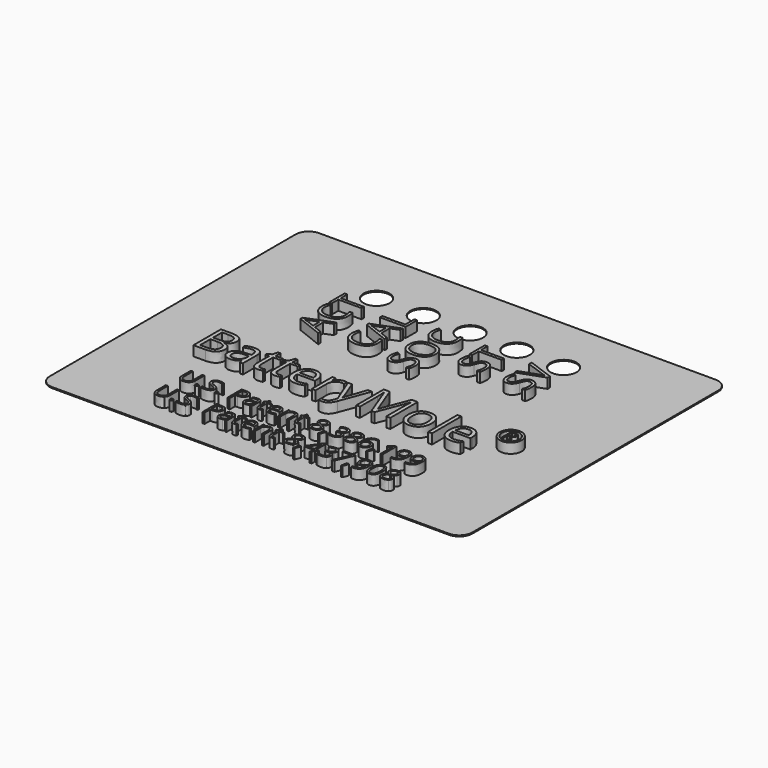
from build123d import *

# Parameters (mm, degrees)
F0_R           = 1.5
F2_DEPTH       = 0.127
F1_R           = 1.27
F1_R_2         = 1.016
F1_TEXT_SIZE   = 4.1666666667
F1_TEXT_SIZE_2 = 5.5555555556
F1_TEXT_SIZE_3 = 2.0717814957
F1_TEXT_SIZE_4 = 2.8222222222
F3_DEPTH       = 1.27


# Not quite as in the source:
# - Text() gives the source's letters only with a copy of the font that has no kerning and outlines rounded to 1/6400 em; it was checked with that copy


with BuildPart() as f2:
    # F0 (on Top) → F2 (new body)
    with BuildSketch(Plane.XY):
        with BuildLine():
            Line((47.3, 38.5), (1.5, 38.5))
            ThreePointArc((1.5, 38.5), (0.4393398282, 38.0606601718), (0, 37))
            Line((0, 37), (0, 1.5))
            ThreePointArc((0, 1.5), (0.4393398282, 0.4393398282), (1.5, 0))
            Line((1.5, 0), (47.3, 0))
            ThreePointArc((47.3, 0), (48.3606601718, 0.4393398282), (48.8, 1.5))
            Line((48.8, 1.5), (48.8, 37))
            ThreePointArc((48.8, 37), (48.3606601718, 38.0606601718), (47.3, 38.5))
        make_face()
        with Locations((13.5, 31.8)):
            Circle(F0_R, mode=Mode.SUBTRACT)
        with Locations((18.9, 31.8)):
            Circle(F0_R, mode=Mode.SUBTRACT)
        with Locations((24.3, 31.8)):
            Circle(F0_R, mode=Mode.SUBTRACT)
        with Locations((29.7, 31.8)):
            Circle(F0_R, mode=Mode.SUBTRACT)
        with Locations((35.1, 31.8)):
            Circle(F0_R, mode=Mode.SUBTRACT)
    extrude(amount=F2_DEPTH)

    # F1 (on Top) → F3 (join)
    with BuildSketch(Plane.XY):
        with Locations((41.1306089235, 16.6292472288)):
            Circle(F1_R)
        with Locations((41.1306089235, 16.6292472288)):
            Circle(F1_R_2, mode=Mode.SUBTRACT)
        with BuildLine():
            add(Edge.make_bspline(
                [(36.4412881944, 3.9645432287), (36.4412881944, 3.4419911453), (36.2765850694, 3.1842428814)],
                knots=[0, 0, 0, 1, 1, 1], degree=2))
            add(Edge.make_bspline(
                [(36.2710729167, 4.7347012148), (36.4412881944, 4.4685744787), (36.4412881944, 3.9645432287)],
                knots=[0, 0, 0, 1, 1, 1], degree=2))
            add(Edge.make_bspline(
                [(35.7727743056, 5.0008279509), (36.1008576389, 5.0008279509), (36.2710729167, 4.7347012148)],
                knots=[0, 0, 0, 1, 1, 1], degree=2))
            add(Edge.make_bspline(
                [(35.2727118056, 4.7457255203), (35.4367534722, 5.0008279509), (35.7727743056, 5.0008279509)],
                knots=[0, 0, 0, 1, 1, 1], degree=2))
            add(Edge.make_bspline(
                [(35.1086701389, 3.9645432287), (35.1086701389, 4.4906230898), (35.2727118056, 4.7457255203)],
                knots=[0, 0, 0, 1, 1, 1], degree=2))
            add(Edge.make_bspline(
                [(35.2782239583, 3.1904164925), (35.1086701389, 3.4543383675), (35.1086701389, 3.9645432287)],
                knots=[0, 0, 0, 1, 1, 1], degree=2))
            add(Edge.make_bspline(
                [(35.7727743056, 2.9264946175), (35.4477777778, 2.9264946175), (35.2782239583, 3.1904164925)],
                knots=[0, 0, 0, 1, 1, 1], degree=2))
            add(Edge.make_bspline(
                [(36.2765850694, 3.1842428814), (36.1118819444, 2.9264946175), (35.7727743056, 2.9264946175)],
                knots=[0, 0, 0, 1, 1, 1], degree=2))
        make_face()
        with BuildLine():
            add(Edge.make_bspline(
                [(35.3401805556, 3.9645432287), (35.3401805556, 3.5248939231), (35.4435885417, 3.324251562)],
                knots=[0, 0, 0, 1, 1, 1], degree=2))
            add(Edge.make_bspline(
                [(35.4435885417, 4.6032914925), (35.3401805556, 4.4041925342), (35.3401805556, 3.9645432287)],
                knots=[0, 0, 0, 1, 1, 1], degree=2))
            add(Edge.make_bspline(
                [(35.7727743056, 4.8023904509), (35.5469965278, 4.8023904509), (35.4435885417, 4.6032914925)],
                knots=[0, 0, 0, 1, 1, 1], degree=2))
            add(Edge.make_bspline(
                [(36.1041649306, 4.6004251731), (36.0016388889, 4.8023904509), (35.7727743056, 4.8023904509)],
                knots=[0, 0, 0, 1, 1, 1], degree=2))
            add(Edge.make_bspline(
                [(36.2066909722, 3.9645432287), (36.2066909722, 4.3984598953), (36.1041649306, 4.6004251731)],
                knots=[0, 0, 0, 1, 1, 1], degree=2))
            add(Edge.make_bspline(
                [(36.1041649306, 3.3268973953), (36.2066909722, 3.5301855898), (36.2066909722, 3.9645432287)],
                knots=[0, 0, 0, 1, 1, 1], degree=2))
            add(Edge.make_bspline(
                [(35.7727743056, 3.1236092009), (36.0016388889, 3.1236092009), (36.1041649306, 3.3268973953)],
                knots=[0, 0, 0, 1, 1, 1], degree=2))
            add(Edge.make_bspline(
                [(35.4435885417, 3.324251562), (35.5469965278, 3.1236092009), (35.7727743056, 3.1236092009)],
                knots=[0, 0, 0, 1, 1, 1], degree=2))
        make_face(mode=Mode.SUBTRACT)
        with BuildLine():
            add(Edge.make_bspline(
                [(37.3862916667, 4.9977411453), (37.6618993056, 4.9977411453), (37.8230746528, 4.8696387148)],
                knots=[0, 0, 0, 1, 1, 1], degree=2))
            add(Edge.make_bspline(
                [(36.9528159722, 4.8676543398), (37.1146527778, 4.9977411453), (37.3862916667, 4.9977411453)],
                knots=[0, 0, 0, 1, 1, 1], degree=2))
            add(Edge.make_bspline(
                [(36.7909791667, 4.5184043398), (36.7909791667, 4.7375675342), (36.9528159722, 4.8676543398)],
                knots=[0, 0, 0, 1, 1, 1], degree=2))
            add(Edge.make_bspline(
                [(36.8736614583, 4.2392689231), (36.7909791667, 4.364064062), (36.7909791667, 4.5184043398)],
                knots=[0, 0, 0, 1, 1, 1], degree=2))
            add(Edge.make_bspline(
                [(37.1464027778, 4.0073175342), (36.95634375, 4.1144737842), (36.8736614583, 4.2392689231)],
                knots=[0, 0, 0, 1, 1, 1], degree=2))
            add(Edge.make_bspline(
                [(36.7248333333, 3.4684494787), (36.7248333333, 3.8141717009), (37.1464027778, 4.0073175342)],
                knots=[0, 0, 0, 1, 1, 1], degree=2))
            add(Edge.make_bspline(
                [(36.8985763889, 3.0678262148), (36.7248333333, 3.209157812), (36.7248333333, 3.4684494787)],
                knots=[0, 0, 0, 1, 1, 1], degree=2))
            add(Edge.make_bspline(
                [(37.3946701389, 2.9264946175), (37.0723194444, 2.9264946175), (36.8985763889, 3.0678262148)],
                knots=[0, 0, 0, 1, 1, 1], degree=2))
            add(Edge.make_bspline(
                [(37.8740069444, 3.076204687), (37.6989409722, 2.9264946175), (37.3946701389, 2.9264946175)],
                knots=[0, 0, 0, 1, 1, 1], degree=2))
            add(Edge.make_bspline(
                [(38.0490729167, 3.4763869787), (38.0490729167, 3.2259147564), (37.8740069444, 3.076204687)],
                knots=[0, 0, 0, 1, 1, 1], degree=2))
            add(Edge.make_bspline(
                [(37.9456649306, 3.7749251731), (38.0490729167, 3.6461612842), (38.0490729167, 3.4763869787)],
                knots=[0, 0, 0, 1, 1, 1], degree=2))
            add(Edge.make_bspline(
                [(37.5970763889, 4.0209876731), (37.8422569444, 3.903689062), (37.9456649306, 3.7749251731)],
                knots=[0, 0, 0, 1, 1, 1], degree=2))
            add(Edge.make_bspline(
                [(37.8920868056, 4.2441196175), (37.7999236111, 4.1215293398), (37.5970763889, 4.0209876731)],
                knots=[0, 0, 0, 1, 1, 1], degree=2))
            add(Edge.make_bspline(
                [(37.98425, 4.5157585064), (37.98425, 4.3667098953), (37.8920868056, 4.2441196175)],
                knots=[0, 0, 0, 1, 1, 1], degree=2))
            add(Edge.make_bspline(
                [(37.8230746528, 4.8696387148), (37.98425, 4.7415362842), (37.98425, 4.5157585064)],
                knots=[0, 0, 0, 1, 1, 1], degree=2))
        make_face()
        with BuildLine():
            add(Edge.make_bspline(
                [(36.9510520833, 3.4627168398), (36.9510520833, 3.2973522564), (37.0659253472, 3.2049685759)],
                knots=[0, 0, 0, 1, 1, 1], degree=2))
            add(Edge.make_bspline(
                [(37.0432152778, 3.7184807287), (36.9510520833, 3.6117654509), (36.9510520833, 3.4627168398)],
                knots=[0, 0, 0, 1, 1, 1], degree=2))
            add(Edge.make_bspline(
                [(37.3408715278, 3.9133904509), (37.1353784722, 3.8251960064), (37.0432152778, 3.7184807287)],
                knots=[0, 0, 0, 1, 1, 1], degree=2))
            add(Edge.make_bspline(
                [(37.7156979167, 3.7114251731), (37.6081006944, 3.8154946175), (37.3408715278, 3.9133904509)],
                knots=[0, 0, 0, 1, 1, 1], degree=2))
            add(Edge.make_bspline(
                [(37.8232951389, 3.4737411453), (37.8232951389, 3.6073557287), (37.7156979167, 3.7114251731)],
                knots=[0, 0, 0, 1, 1, 1], degree=2))
            add(Edge.make_bspline(
                [(37.7088628472, 3.209157812), (37.8232951389, 3.3057307287), (37.8232951389, 3.4737411453)],
                knots=[0, 0, 0, 1, 1, 1], degree=2))
            add(Edge.make_bspline(
                [(37.3889375, 3.1125848953), (37.5944305556, 3.1125848953), (37.7088628472, 3.209157812)],
                knots=[0, 0, 0, 1, 1, 1], degree=2))
            add(Edge.make_bspline(
                [(37.0659253472, 3.2049685759), (37.1807986111, 3.1125848953), (37.3889375, 3.1125848953)],
                knots=[0, 0, 0, 1, 1, 1], degree=2))
        make_face(mode=Mode.SUBTRACT)
        with BuildLine():
            add(Edge.make_bspline(
                [(37.3836458333, 4.8120918398), (37.2112256944, 4.8120918398), (37.1133298611, 4.7294095481)],
                knots=[0, 0, 0, 1, 1, 1], degree=2))
            add(Edge.make_bspline(
                [(37.6585920139, 4.7300710064), (37.5587118056, 4.8120918398), (37.3836458333, 4.8120918398)],
                knots=[0, 0, 0, 1, 1, 1], degree=2))
            add(Edge.make_bspline(
                [(37.7584722222, 4.5087029509), (37.7584722222, 4.6480501731), (37.6585920139, 4.7300710064)],
                knots=[0, 0, 0, 1, 1, 1], degree=2))
            add(Edge.make_bspline(
                [(37.6764513889, 4.2868939231), (37.7584722222, 4.3821439231), (37.7584722222, 4.5087029509)],
                knots=[0, 0, 0, 1, 1, 1], degree=2))
            add(Edge.make_bspline(
                [(37.3973159722, 4.1091821175), (37.5944305556, 4.1916439231), (37.6764513889, 4.2868939231)],
                knots=[0, 0, 0, 1, 1, 1], degree=2))
            add(Edge.make_bspline(
                [(37.0967934028, 4.2910831592), (37.1781527778, 4.2000223953), (37.3973159722, 4.1091821175)],
                knots=[0, 0, 0, 1, 1, 1], degree=2))
            add(Edge.make_bspline(
                [(37.0154340278, 4.5087029509), (37.0154340278, 4.3821439231), (37.0967934028, 4.2910831592)],
                knots=[0, 0, 0, 1, 1, 1], degree=2))
            add(Edge.make_bspline(
                [(37.1133298611, 4.7294095481), (37.0154340278, 4.6467272564), (37.0154340278, 4.5087029509)],
                knots=[0, 0, 0, 1, 1, 1], degree=2))
        make_face(mode=Mode.SUBTRACT)
        with BuildLine():
            add(Edge.make_bspline(
                [(26.3214166667, 4.9977411453), (26.5970243056, 4.9977411453), (26.7581996528, 4.8696387148)],
                knots=[0, 0, 0, 1, 1, 1], degree=2))
            add(Edge.make_bspline(
                [(25.8879409722, 4.8676543398), (26.0497777778, 4.9977411453), (26.3214166667, 4.9977411453)],
                knots=[0, 0, 0, 1, 1, 1], degree=2))
            add(Edge.make_bspline(
                [(25.7261041667, 4.5184043398), (25.7261041667, 4.7375675342), (25.8879409722, 4.8676543398)],
                knots=[0, 0, 0, 1, 1, 1], degree=2))
            add(Edge.make_bspline(
                [(25.8087864583, 4.2392689231), (25.7261041667, 4.364064062), (25.7261041667, 4.5184043398)],
                knots=[0, 0, 0, 1, 1, 1], degree=2))
            add(Edge.make_bspline(
                [(26.0815277778, 4.0073175342), (25.89146875, 4.1144737842), (25.8087864583, 4.2392689231)],
                knots=[0, 0, 0, 1, 1, 1], degree=2))
            add(Edge.make_bspline(
                [(25.6599583333, 3.4684494787), (25.6599583333, 3.8141717009), (26.0815277778, 4.0073175342)],
                knots=[0, 0, 0, 1, 1, 1], degree=2))
            add(Edge.make_bspline(
                [(25.8337013889, 3.0678262148), (25.6599583333, 3.209157812), (25.6599583333, 3.4684494787)],
                knots=[0, 0, 0, 1, 1, 1], degree=2))
            add(Edge.make_bspline(
                [(26.3297951389, 2.9264946175), (26.0074444444, 2.9264946175), (25.8337013889, 3.0678262148)],
                knots=[0, 0, 0, 1, 1, 1], degree=2))
            add(Edge.make_bspline(
                [(26.8091319444, 3.076204687), (26.6340659722, 2.9264946175), (26.3297951389, 2.9264946175)],
                knots=[0, 0, 0, 1, 1, 1], degree=2))
            add(Edge.make_bspline(
                [(26.9841979167, 3.4763869787), (26.9841979167, 3.2259147564), (26.8091319444, 3.076204687)],
                knots=[0, 0, 0, 1, 1, 1], degree=2))
            add(Edge.make_bspline(
                [(26.8807899306, 3.7749251731), (26.9841979167, 3.6461612842), (26.9841979167, 3.4763869787)],
                knots=[0, 0, 0, 1, 1, 1], degree=2))
            add(Edge.make_bspline(
                [(26.5322013889, 4.0209876731), (26.7773819444, 3.903689062), (26.8807899306, 3.7749251731)],
                knots=[0, 0, 0, 1, 1, 1], degree=2))
            add(Edge.make_bspline(
                [(26.8272118056, 4.2441196175), (26.7350486111, 4.1215293398), (26.5322013889, 4.0209876731)],
                knots=[0, 0, 0, 1, 1, 1], degree=2))
            add(Edge.make_bspline(
                [(26.919375, 4.5157585064), (26.919375, 4.3667098953), (26.8272118056, 4.2441196175)],
                knots=[0, 0, 0, 1, 1, 1], degree=2))
            add(Edge.make_bspline(
                [(26.7581996528, 4.8696387148), (26.919375, 4.7415362842), (26.919375, 4.5157585064)],
                knots=[0, 0, 0, 1, 1, 1], degree=2))
        make_face()
        with BuildLine():
            add(Edge.make_bspline(
                [(25.8861770833, 3.4627168398), (25.8861770833, 3.2973522564), (26.0010503472, 3.2049685759)],
                knots=[0, 0, 0, 1, 1, 1], degree=2))
            add(Edge.make_bspline(
                [(25.9783402778, 3.7184807287), (25.8861770833, 3.6117654509), (25.8861770833, 3.4627168398)],
                knots=[0, 0, 0, 1, 1, 1], degree=2))
            add(Edge.make_bspline(
                [(26.2759965278, 3.9133904509), (26.0705034722, 3.8251960064), (25.9783402778, 3.7184807287)],
                knots=[0, 0, 0, 1, 1, 1], degree=2))
            add(Edge.make_bspline(
                [(26.6508229167, 3.7114251731), (26.5432256944, 3.8154946175), (26.2759965278, 3.9133904509)],
                knots=[0, 0, 0, 1, 1, 1], degree=2))
            add(Edge.make_bspline(
                [(26.7584201389, 3.4737411453), (26.7584201389, 3.6073557287), (26.6508229167, 3.7114251731)],
                knots=[0, 0, 0, 1, 1, 1], degree=2))
            add(Edge.make_bspline(
                [(26.6439878472, 3.209157812), (26.7584201389, 3.3057307287), (26.7584201389, 3.4737411453)],
                knots=[0, 0, 0, 1, 1, 1], degree=2))
            add(Edge.make_bspline(
                [(26.3240625, 3.1125848953), (26.5295555556, 3.1125848953), (26.6439878472, 3.209157812)],
                knots=[0, 0, 0, 1, 1, 1], degree=2))
            add(Edge.make_bspline(
                [(26.0010503472, 3.2049685759), (26.1159236111, 3.1125848953), (26.3240625, 3.1125848953)],
                knots=[0, 0, 0, 1, 1, 1], degree=2))
        make_face(mode=Mode.SUBTRACT)
        with BuildLine():
            add(Edge.make_bspline(
                [(26.3187708333, 4.8120918398), (26.1463506944, 4.8120918398), (26.0484548611, 4.7294095481)],
                knots=[0, 0, 0, 1, 1, 1], degree=2))
            add(Edge.make_bspline(
                [(26.5937170139, 4.7300710064), (26.4938368056, 4.8120918398), (26.3187708333, 4.8120918398)],
                knots=[0, 0, 0, 1, 1, 1], degree=2))
            add(Edge.make_bspline(
                [(26.6935972222, 4.5087029509), (26.6935972222, 4.6480501731), (26.5937170139, 4.7300710064)],
                knots=[0, 0, 0, 1, 1, 1], degree=2))
            add(Edge.make_bspline(
                [(26.6115763889, 4.2868939231), (26.6935972222, 4.3821439231), (26.6935972222, 4.5087029509)],
                knots=[0, 0, 0, 1, 1, 1], degree=2))
            add(Edge.make_bspline(
                [(26.3324409722, 4.1091821175), (26.5295555556, 4.1916439231), (26.6115763889, 4.2868939231)],
                knots=[0, 0, 0, 1, 1, 1], degree=2))
            add(Edge.make_bspline(
                [(26.0319184028, 4.2910831592), (26.1132777778, 4.2000223953), (26.3324409722, 4.1091821175)],
                knots=[0, 0, 0, 1, 1, 1], degree=2))
            add(Edge.make_bspline(
                [(25.9505590278, 4.5087029509), (25.9505590278, 4.3821439231), (26.0319184028, 4.2910831592)],
                knots=[0, 0, 0, 1, 1, 1], degree=2))
            add(Edge.make_bspline(
                [(26.0484548611, 4.7294095481), (25.9505590278, 4.6467272564), (25.9505590278, 4.5087029509)],
                knots=[0, 0, 0, 1, 1, 1], degree=2))
        make_face(mode=Mode.SUBTRACT)
        with Locations(Location((36.6, 24.262890625), (0, 0, 90))):
            Text('SV', F1_TEXT_SIZE, font='Open Sans', text_align=(TextAlign.LEFT, TextAlign.BOTTOM))
        with Locations(Location((25.8, 20.993359375), (0, 0, 90))):
            Text('SOC', F1_TEXT_SIZE, font='Open Sans', text_align=(TextAlign.LEFT, TextAlign.BOTTOM))
        with Locations((7.1502256944, 12.6292472288)):
            Text('BatteryMole', F1_TEXT_SIZE_2, font='Open Sans', text_align=(TextAlign.LEFT, TextAlign.BOTTOM))
        with BuildLine():
            add(Edge.make_bspline(
                [(34.8167465278, 4.1091821175), (34.8167465278, 2.9264946175), (33.9017291667, 2.9264946175)],
                knots=[0, 0, 0, 1, 1, 1], degree=2))
            add(Edge.make_bspline(
                [(34.7340642361, 4.5852116314), (34.8167465278, 4.3834668398), (34.8167465278, 4.1091821175)],
                knots=[0, 0, 0, 1, 1, 1], degree=2))
            add(Edge.make_bspline(
                [(34.497703125, 4.8923487842), (34.6513819444, 4.7869564231), (34.7340642361, 4.5852116314)],
                knots=[0, 0, 0, 1, 1, 1], degree=2))
            add(Edge.make_bspline(
                [(34.13853125, 4.9977411453), (34.3440243056, 4.9977411453), (34.497703125, 4.8923487842)],
                knots=[0, 0, 0, 1, 1, 1], degree=2))
            add(Edge.make_bspline(
                [(33.676171875, 4.8158401037), (33.8518993056, 4.9977411453), (34.13853125, 4.9977411453)],
                knots=[0, 0, 0, 1, 1, 1], degree=2))
            add(Edge.make_bspline(
                [(33.5004444444, 4.3199668398), (33.5004444444, 4.633939062), (33.676171875, 4.8158401037)],
                knots=[0, 0, 0, 1, 1, 1], degree=2))
            add(Edge.make_bspline(
                [(33.6576510417, 3.8734824648), (33.5004444444, 4.0333348953), (33.5004444444, 4.3199668398)],
                knots=[0, 0, 0, 1, 1, 1], degree=2))
            add(Edge.make_bspline(
                [(34.0820868056, 3.7136300342), (33.8148576389, 3.7136300342), (33.6576510417, 3.8734824648)],
                knots=[0, 0, 0, 1, 1, 1], degree=2))
            add(Edge.make_bspline(
                [(34.3645295139, 3.7736022564), (34.2390729167, 3.7136300342), (34.0820868056, 3.7136300342)],
                knots=[0, 0, 0, 1, 1, 1], degree=2))
            add(Edge.make_bspline(
                [(34.5658333333, 3.9477862842), (34.4899861111, 3.8335744787), (34.3645295139, 3.7736022564)],
                knots=[0, 0, 0, 1, 1, 1], degree=2))
            Line((34.5658333333, 3.9477862842), (34.5821493056, 3.9477862842))
            add(Edge.make_bspline(
                [(34.3982638889, 3.320282812), (34.56715625, 3.5248939231), (34.5821493056, 3.9477862842)],
                knots=[0, 0, 0, 1, 1, 1], degree=2))
            add(Edge.make_bspline(
                [(33.8986423611, 3.1156717009), (34.2293715278, 3.1156717009), (34.3982638889, 3.320282812)],
                knots=[0, 0, 0, 1, 1, 1], degree=2))
            add(Edge.make_bspline(
                [(33.6481701389, 3.1513904509), (33.7584131944, 3.1156717009), (33.8986423611, 3.1156717009)],
                knots=[0, 0, 0, 1, 1, 1], degree=2))
            Line((33.6481701389, 3.1513904509), (33.6481701389, 2.9542758675))
            add(Edge.make_bspline(
                [(33.9017291667, 2.9264946175), (33.74165625, 2.9264946175), (33.6481701389, 2.9542758675)],
                knots=[0, 0, 0, 1, 1, 1], degree=2))
        make_face()
        with BuildLine():
            add(Edge.make_bspline(
                [(34.13853125, 4.8023904509), (33.9414166667, 4.8023904509), (33.8340399306, 4.675610937)],
                knots=[0, 0, 0, 1, 1, 1], degree=2))
            add(Edge.make_bspline(
                [(34.370703125, 4.7320553814), (34.2695, 4.8023904509), (34.13853125, 4.8023904509)],
                knots=[0, 0, 0, 1, 1, 1], degree=2))
            add(Edge.make_bspline(
                [(34.5285711806, 4.5391300342), (34.47190625, 4.661720312), (34.370703125, 4.7320553814)],
                knots=[0, 0, 0, 1, 1, 1], degree=2))
            add(Edge.make_bspline(
                [(34.5852361111, 4.2719008675), (34.5852361111, 4.4165397564), (34.5285711806, 4.5391300342)],
                knots=[0, 0, 0, 1, 1, 1], degree=2))
            add(Edge.make_bspline(
                [(34.5246024306, 4.0871335064), (34.5852361111, 4.1753279509), (34.5852361111, 4.2719008675)],
                knots=[0, 0, 0, 1, 1, 1], degree=2))
            add(Edge.make_bspline(
                [(34.3585763889, 3.9480067703), (34.46396875, 3.998939062), (34.5246024306, 4.0871335064)],
                knots=[0, 0, 0, 1, 1, 1], degree=2))
            add(Edge.make_bspline(
                [(34.1275069444, 3.8970744787), (34.2531840278, 3.8970744787), (34.3585763889, 3.9480067703)],
                knots=[0, 0, 0, 1, 1, 1], degree=2))
            add(Edge.make_bspline(
                [(33.8258819444, 4.0106248259), (33.9251006944, 3.8970744787), (34.1275069444, 3.8970744787)],
                knots=[0, 0, 0, 1, 1, 1], degree=2))
            add(Edge.make_bspline(
                [(33.7266631944, 4.3226126731), (33.7266631944, 4.1241751731), (33.8258819444, 4.0106248259)],
                knots=[0, 0, 0, 1, 1, 1], degree=2))
            add(Edge.make_bspline(
                [(33.8340399306, 4.675610937), (33.7266631944, 4.5488314231), (33.7266631944, 4.3226126731)],
                knots=[0, 0, 0, 1, 1, 1], degree=2))
        make_face(mode=Mode.SUBTRACT)
        with Locations(Location((31.2, 24.4764322917), (0, 0, 90))):
            Text('ST', F1_TEXT_SIZE, font='Open Sans', text_align=(TextAlign.LEFT, TextAlign.BOTTOM))
        with Locations(Location((15, 21.4979166667), (0, 0, 90))):
            Text('ACT', F1_TEXT_SIZE, font='Open Sans', text_align=(TextAlign.LEFT, TextAlign.BOTTOM))
        with BuildLine():
            add(Edge.make_bspline(
                [(17.7612638889, 4.3821439231), (17.7612638889, 4.0761092009), (17.5524635417, 3.9114060759)],
                knots=[0, 0, 0, 1, 1, 1], degree=2))
            add(Edge.make_bspline(
                [(17.0063194444, 4.9690779509), (17.7612638889, 4.9690779509), (17.7612638889, 4.3821439231)],
                knots=[0, 0, 0, 1, 1, 1], degree=2))
            Line((17.0063194444, 4.9690779509), (16.4837673611, 4.9690779509))
            Line((16.4837673611, 4.9690779509), (16.4837673611, 2.9542758675))
            Line((16.4837673611, 2.9542758675), (16.7179236111, 2.9542758675))
            Line((16.7179236111, 2.9542758675), (16.7179236111, 3.7467029509))
            Line((16.7179236111, 3.7467029509), (16.9551666667, 3.7467029509))
            add(Edge.make_bspline(
                [(17.5524635417, 3.9114060759), (17.3436631944, 3.7467029509), (16.9551666667, 3.7467029509)],
                knots=[0, 0, 0, 1, 1, 1], degree=2))
        make_face()
        with BuildLine():
            Line((16.9291493056, 3.9477862842), (16.7179236111, 3.9477862842))
            Line((16.7179236111, 3.9477862842), (16.7179236111, 4.7662307287))
            Line((16.7179236111, 4.7662307287), (16.9798611111, 4.7662307287))
            add(Edge.make_bspline(
                [(17.3877604167, 4.6685553814), (17.2567916667, 4.7662307287), (16.9798611111, 4.7662307287)],
                knots=[0, 0, 0, 1, 1, 1], degree=2))
            add(Edge.make_bspline(
                [(17.5187291667, 4.3711196175), (17.5187291667, 4.5708800342), (17.3877604167, 4.6685553814)],
                knots=[0, 0, 0, 1, 1, 1], degree=2))
            add(Edge.make_bspline(
                [(17.3796024306, 4.0483279509), (17.5187291667, 4.1488696175), (17.5187291667, 4.3711196175)],
                knots=[0, 0, 0, 1, 1, 1], degree=2))
            add(Edge.make_bspline(
                [(16.9291493056, 3.9477862842), (17.2404756944, 3.9477862842), (17.3796024306, 4.0483279509)],
                knots=[0, 0, 0, 1, 1, 1], degree=2))
        make_face(mode=Mode.SUBTRACT)
        with Locations(Location((20.4, 21.6971354167), (0, 0, 90))):
            Text('CAL', F1_TEXT_SIZE, font='Open Sans', text_align=(TextAlign.LEFT, TextAlign.BOTTOM))
        Polygon((29.0801388889, 3.4172967009), (29.3791180556, 3.4172967009), (29.3791180556, 3.6254355898), (29.0801388889, 3.6254355898), (29.0801388889, 4.9801022564), (28.8376041667, 4.9801022564), (27.8811354167, 3.6170571175), (27.8811354167, 3.4172967009), (28.8609756944, 3.4172967009), (28.8609756944, 2.9542758675), (29.0801388889, 2.9542758675), align=None)
        with BuildLine():
            Line((28.8609756944, 4.2952723953), (28.8609756944, 3.6254355898))
            Line((28.8609756944, 3.6254355898), (28.11, 3.6254355898))
            Line((28.11, 3.6254355898), (28.7397083333, 4.5210501731))
            add(Edge.make_bspline(
                [(28.8640625, 4.7402133675), (28.7979166667, 4.6079217009), (28.7397083333, 4.5210501731)],
                knots=[0, 0, 0, 1, 1, 1], degree=2))
            Line((28.8640625, 4.7402133675), (28.8750868056, 4.7402133675))
            add(Edge.make_bspline(
                [(28.8609756944, 4.2952723953), (28.8609756944, 4.4923869787), (28.8750868056, 4.7402133675)],
                knots=[0, 0, 0, 1, 1, 1], degree=2))
        make_face(mode=Mode.SUBTRACT)
        with BuildLine():
            Line((19.0317048611, 3.169470312), (19.077125, 2.9542758675))
            Line((19.077125, 2.9542758675), (19.2468993056, 2.9542758675))
            Line((19.2468993056, 2.9542758675), (19.2468993056, 3.9852689231))
            add(Edge.make_bspline(
                [(19.1165920139, 4.3695762148), (19.2468993056, 4.2498522564), (19.2468993056, 3.9852689231)],
                knots=[0, 0, 0, 1, 1, 1], degree=2))
            add(Edge.make_bspline(
                [(18.7164097222, 4.4893001731), (18.9862847222, 4.4893001731), (19.1165920139, 4.3695762148)],
                knots=[0, 0, 0, 1, 1, 1], degree=2))
            add(Edge.make_bspline(
                [(18.4494010417, 4.4549043398), (18.5823541667, 4.4893001731), (18.7164097222, 4.4893001731)],
                knots=[0, 0, 0, 1, 1, 1], degree=2))
            add(Edge.make_bspline(
                [(18.2048819444, 4.360095312), (18.3164479167, 4.4205085064), (18.4494010417, 4.4549043398)],
                knots=[0, 0, 0, 1, 1, 1], degree=2))
            Line((18.2048819444, 4.360095312), (18.2754375, 4.1850293398))
            add(Edge.make_bspline(
                [(18.7022986111, 4.300564062), (18.5135625, 4.300564062), (18.2754375, 4.1850293398)],
                knots=[0, 0, 0, 1, 1, 1], degree=2))
            add(Edge.make_bspline(
                [(18.9470381944, 4.2158973953), (18.87075, 4.300564062), (18.7022986111, 4.300564062)],
                knots=[0, 0, 0, 1, 1, 1], degree=2))
            add(Edge.make_bspline(
                [(19.0233263889, 3.9535189231), (19.0233263889, 4.1312307287), (18.9470381944, 4.2158973953)],
                knots=[0, 0, 0, 1, 1, 1], degree=2))
            Line((19.0233263889, 3.9535189231), (19.0233263889, 3.8595918398))
            Line((19.0233263889, 3.8595918398), (18.7671215278, 3.8512133675))
            add(Edge.make_bspline(
                [(18.0355486111, 3.371876562), (18.0355486111, 3.8291647564), (18.7671215278, 3.8512133675)],
                knots=[0, 0, 0, 1, 1, 1], degree=2))
            add(Edge.make_bspline(
                [(18.1629895833, 3.042470312), (18.0355486111, 3.1584460064), (18.0355486111, 3.371876562)],
                knots=[0, 0, 0, 1, 1, 1], degree=2))
            add(Edge.make_bspline(
                [(18.5148854167, 2.9264946175), (18.2904305556, 2.9264946175), (18.1629895833, 3.042470312)],
                knots=[0, 0, 0, 1, 1, 1], degree=2))
            add(Edge.make_bspline(
                [(18.7955642361, 2.976985937), (18.6833368056, 2.9264946175), (18.5148854167, 2.9264946175)],
                knots=[0, 0, 0, 1, 1, 1], degree=2))
            add(Edge.make_bspline(
                [(19.0206805556, 3.169470312), (18.9077916667, 3.0274772564), (18.7955642361, 2.976985937)],
                knots=[0, 0, 0, 1, 1, 1], degree=2))
            Line((19.0206805556, 3.169470312), (19.0317048611, 3.169470312))
        make_face()
        with BuildLine():
            add(Edge.make_bspline(
                [(18.5603055556, 3.1156717009), (18.7741770833, 3.1156717009), (18.8961059028, 3.2327498259)],
                knots=[0, 0, 0, 1, 1, 1], degree=2))
            add(Edge.make_bspline(
                [(18.3504027778, 3.1802741314), (18.4253680556, 3.1156717009), (18.5603055556, 3.1156717009)],
                knots=[0, 0, 0, 1, 1, 1], degree=2))
            add(Edge.make_bspline(
                [(18.2754375, 3.3692307287), (18.2754375, 3.244876562), (18.3504027778, 3.1802741314)],
                knots=[0, 0, 0, 1, 1, 1], degree=2))
            add(Edge.make_bspline(
                [(18.3958229167, 3.6027255203), (18.2754375, 3.5275397564), (18.2754375, 3.3692307287)],
                knots=[0, 0, 0, 1, 1, 1], degree=2))
            add(Edge.make_bspline(
                [(18.7891701389, 3.6876126731), (18.5162083333, 3.6779112842), (18.3958229167, 3.6027255203)],
                knots=[0, 0, 0, 1, 1, 1], degree=2))
            Line((18.7891701389, 3.6876126731), (19.0180347222, 3.6968730898))
            Line((19.0180347222, 3.6968730898), (19.0180347222, 3.5606126731))
            add(Edge.make_bspline(
                [(18.8961059028, 3.2327498259), (19.0180347222, 3.3498279509), (19.0180347222, 3.5606126731)],
                knots=[0, 0, 0, 1, 1, 1], degree=2))
        make_face(mode=Mode.SUBTRACT)
        with BuildLine():
            add(Edge.make_bspline(
                [(21.3521006944, 2.9264946175), (21.0174027778, 2.9264946175), (20.8235954861, 3.1306647564)],
                knots=[0, 0, 0, 1, 1, 1], degree=2))
            add(Edge.make_bspline(
                [(21.61315625, 2.9494251731), (21.5051180556, 2.9264946175), (21.3521006944, 2.9264946175)],
                knots=[0, 0, 0, 1, 1, 1], degree=2))
            add(Edge.make_bspline(
                [(21.8424618056, 3.0243904509), (21.7211944444, 2.9723557287), (21.61315625, 2.9494251731)],
                knots=[0, 0, 0, 1, 1, 1], degree=2))
            Line((21.8424618056, 3.0243904509), (21.8424618056, 3.2285605898))
            add(Edge.make_bspline(
                [(21.3604791667, 3.1266960064), (21.6043368056, 3.1266960064), (21.8424618056, 3.2285605898)],
                knots=[0, 0, 0, 1, 1, 1], degree=2))
            add(Edge.make_bspline(
                [(21.0015277778, 3.2644998259), (21.12896875, 3.1266960064), (21.3604791667, 3.1266960064)],
                knots=[0, 0, 0, 1, 1, 1], degree=2))
            add(Edge.make_bspline(
                [(20.86703125, 3.6682098953), (20.8740868056, 3.4023036453), (21.0015277778, 3.2644998259)],
                knots=[0, 0, 0, 1, 1, 1], degree=2))
            Line((20.86703125, 3.6682098953), (21.9072847222, 3.6682098953))
            Line((21.9072847222, 3.6682098953), (21.9072847222, 3.8128487842))
            add(Edge.make_bspline(
                [(21.7419201389, 4.3056352425), (21.9072847222, 4.1188835064), (21.9072847222, 3.8128487842)],
                knots=[0, 0, 0, 1, 1, 1], degree=2))
            add(Edge.make_bspline(
                [(21.2930104167, 4.4923869787), (21.5765555556, 4.4923869787), (21.7419201389, 4.3056352425)],
                knots=[0, 0, 0, 1, 1, 1], degree=2))
            add(Edge.make_bspline(
                [(20.8097048611, 4.2774130203), (20.9896215278, 4.4923869787), (21.2930104167, 4.4923869787)],
                knots=[0, 0, 0, 1, 1, 1], degree=2))
            add(Edge.make_bspline(
                [(20.6297881944, 3.6968730898), (20.6297881944, 4.062439062), (20.8097048611, 4.2774130203)],
                knots=[0, 0, 0, 1, 1, 1], degree=2))
            add(Edge.make_bspline(
                [(20.8235954861, 3.1306647564), (20.6297881944, 3.3348348953), (20.6297881944, 3.6968730898)],
                knots=[0, 0, 0, 1, 1, 1], degree=2))
        make_face()
        with BuildLine():
            add(Edge.make_bspline(
                [(21.2899236111, 4.300564062), (21.1082430556, 4.300564062), (20.999984375, 4.1821630203)],
                knots=[0, 0, 0, 1, 1, 1], degree=2))
            add(Edge.make_bspline(
                [(21.5657517361, 4.185470312), (21.4693993056, 4.300564062), (21.2899236111, 4.300564062)],
                knots=[0, 0, 0, 1, 1, 1], degree=2))
            add(Edge.make_bspline(
                [(21.6621041667, 3.8543001731), (21.6621041667, 4.070376562), (21.5657517361, 4.185470312)],
                knots=[0, 0, 0, 1, 1, 1], degree=2))
            Line((21.6621041667, 3.8543001731), (20.8723229167, 3.8543001731))
            add(Edge.make_bspline(
                [(20.999984375, 4.1821630203), (20.8917256944, 4.0637619787), (20.8723229167, 3.8543001731)],
                knots=[0, 0, 0, 1, 1, 1], degree=2))
        make_face(mode=Mode.SUBTRACT)
        with BuildLine():
            Line((12.1662083333, 3.665564062), (12.1662083333, 4.9690779509))
            Line((12.1662083333, 4.9690779509), (11.9320520833, 4.9690779509))
            Line((11.9320520833, 4.9690779509), (11.9320520833, 3.6571855898))
            add(Edge.make_bspline(
                [(11.7942482639, 3.2678071175), (11.9320520833, 3.403626562), (11.9320520833, 3.6571855898)],
                knots=[0, 0, 0, 1, 1, 1], degree=2))
            add(Edge.make_bspline(
                [(11.4015625, 3.1319876731), (11.6564444444, 3.1319876731), (11.7942482639, 3.2678071175)],
                knots=[0, 0, 0, 1, 1, 1], degree=2))
            add(Edge.make_bspline(
                [(10.9965295139, 3.2671456592), (11.1343333333, 3.1319876731), (11.4015625, 3.1319876731)],
                knots=[0, 0, 0, 1, 1, 1], degree=2))
            add(Edge.make_bspline(
                [(10.8587256944, 3.6545397564), (10.8587256944, 3.4023036453), (10.9965295139, 3.2671456592)],
                knots=[0, 0, 0, 1, 1, 1], degree=2))
            Line((10.8587256944, 3.6545397564), (10.8587256944, 4.9690779509))
            Line((10.8587256944, 4.9690779509), (10.6241284722, 4.9690779509))
            Line((10.6241284722, 4.9690779509), (10.6241284722, 3.6708557287))
            add(Edge.make_bspline(
                [(10.8232274306, 3.1251526037), (10.6241284722, 3.3238105898), (10.6241284722, 3.6708557287)],
                knots=[0, 0, 0, 1, 1, 1], degree=2))
            add(Edge.make_bspline(
                [(11.3861284722, 2.9264946175), (11.0223263889, 2.9264946175), (10.8232274306, 3.1251526037)],
                knots=[0, 0, 0, 1, 1, 1], degree=2))
            add(Edge.make_bspline(
                [(11.9580694444, 3.1236092009), (11.7499305556, 2.9264946175), (11.3861284722, 2.9264946175)],
                knots=[0, 0, 0, 1, 1, 1], degree=2))
            add(Edge.make_bspline(
                [(12.1662083333, 3.665564062), (12.1662083333, 3.3207237842), (11.9580694444, 3.1236092009)],
                knots=[0, 0, 0, 1, 1, 1], degree=2))
        make_face()
        with Locations((40.4480951614, 15.8901806324)):
            Text('R', F1_TEXT_SIZE_3, font='Open Sans', text_align=(TextAlign.LEFT, TextAlign.BOTTOM))
        with BuildLine():
            add(Edge.make_bspline(
                [(30.8219791667, 4.495032812), (30.8219791667, 4.3018869787), (30.7137204861, 4.1792967009)],
                knots=[0, 0, 0, 1, 1, 1], degree=2))
            add(Edge.make_bspline(
                [(30.6592604167, 4.8634651037), (30.8219791667, 4.729189062), (30.8219791667, 4.495032812)],
                knots=[0, 0, 0, 1, 1, 1], degree=2))
            add(Edge.make_bspline(
                [(30.2032951389, 4.9977411453), (30.4965416667, 4.9977411453), (30.6592604167, 4.8634651037)],
                knots=[0, 0, 0, 1, 1, 1], degree=2))
            add(Edge.make_bspline(
                [(29.8619826389, 4.9419581592), (30.0238194444, 4.9977411453), (30.2032951389, 4.9977411453)],
                knots=[0, 0, 0, 1, 1, 1], degree=2))
            add(Edge.make_bspline(
                [(29.5762326389, 4.7882793398), (29.7001458333, 4.8861751731), (29.8619826389, 4.9419581592)],
                knots=[0, 0, 0, 1, 1, 1], degree=2))
            Line((29.5762326389, 4.7882793398), (29.6917673611, 4.633939062))
            add(Edge.make_bspline(
                [(29.9592170139, 4.7664512148), (29.8421388889, 4.7305119787), (29.6917673611, 4.633939062)],
                knots=[0, 0, 0, 1, 1, 1], degree=2))
            add(Edge.make_bspline(
                [(30.2085868056, 4.8023904509), (30.0762951389, 4.8023904509), (29.9592170139, 4.7664512148)],
                knots=[0, 0, 0, 1, 1, 1], degree=2))
            add(Edge.make_bspline(
                [(30.4835329861, 4.7181647564), (30.3823298611, 4.8023904509), (30.2085868056, 4.8023904509)],
                knots=[0, 0, 0, 1, 1, 1], degree=2))
            add(Edge.make_bspline(
                [(30.5847361111, 4.4866543398), (30.5847361111, 4.633939062), (30.4835329861, 4.7181647564)],
                knots=[0, 0, 0, 1, 1, 1], degree=2))
            add(Edge.make_bspline(
                [(30.4469322917, 4.1978175342), (30.5847361111, 4.3018869787), (30.5847361111, 4.4866543398)],
                knots=[0, 0, 0, 1, 1, 1], degree=2))
            add(Edge.make_bspline(
                [(30.0736493056, 4.0937480898), (30.3091284722, 4.0937480898), (30.4469322917, 4.1978175342)],
                knots=[0, 0, 0, 1, 1, 1], degree=2))
            Line((30.0736493056, 4.0937480898), (29.8725659722, 4.0937480898))
            Line((29.8725659722, 4.0937480898), (29.8725659722, 3.8970744787))
            Line((29.8725659722, 3.8970744787), (30.0710034722, 3.8970744787))
            add(Edge.make_bspline(
                [(30.6469131944, 3.5301855898), (30.6469131944, 3.8970744787), (30.0710034722, 3.8970744787)],
                knots=[0, 0, 0, 1, 1, 1], degree=2))
            add(Edge.make_bspline(
                [(30.1248020833, 3.1209633675), (30.6469131944, 3.1209633675), (30.6469131944, 3.5301855898)],
                knots=[0, 0, 0, 1, 1, 1], degree=2))
            add(Edge.make_bspline(
                [(29.84434375, 3.1546977425), (29.9925104167, 3.1209633675), (30.1248020833, 3.1209633675)],
                knots=[0, 0, 0, 1, 1, 1], degree=2))
            add(Edge.make_bspline(
                [(29.5652083333, 3.2532550342), (29.6961770833, 3.1884321175), (29.84434375, 3.1546977425)],
                knots=[0, 0, 0, 1, 1, 1], degree=2))
            Line((29.5652083333, 3.2532550342), (29.5652083333, 3.0354147564))
            add(Edge.make_bspline(
                [(29.8233975694, 2.9507480898), (29.6904444444, 2.975001562), (29.5652083333, 3.0354147564)],
                knots=[0, 0, 0, 1, 1, 1], degree=2))
            add(Edge.make_bspline(
                [(30.1164236111, 2.9264946175), (29.9563506944, 2.9264946175), (29.8233975694, 2.9507480898)],
                knots=[0, 0, 0, 1, 1, 1], degree=2))
            add(Edge.make_bspline(
                [(30.6839548611, 3.0817168398), (30.4841944444, 2.9264946175), (30.1164236111, 2.9264946175)],
                knots=[0, 0, 0, 1, 1, 1], degree=2))
            add(Edge.make_bspline(
                [(30.8837152778, 3.5248939231), (30.8837152778, 3.236939062), (30.6839548611, 3.0817168398)],
                knots=[0, 0, 0, 1, 1, 1], degree=2))
            add(Edge.make_bspline(
                [(30.7666371528, 3.850110937), (30.8837152778, 3.7259772564), (30.8837152778, 3.5248939231)],
                knots=[0, 0, 0, 1, 1, 1], degree=2))
            add(Edge.make_bspline(
                [(30.4070243056, 4.0042307287), (30.6495590278, 3.9742446175), (30.7666371528, 3.850110937)],
                knots=[0, 0, 0, 1, 1, 1], degree=2))
            Line((30.4070243056, 4.0042307287), (30.4070243056, 4.0152550342))
            add(Edge.make_bspline(
                [(30.7137204861, 4.1792967009), (30.6054618056, 4.0567064231), (30.4070243056, 4.0152550342)],
                knots=[0, 0, 0, 1, 1, 1], degree=2))
        make_face()
        with BuildLine():
            add(Edge.make_bspline(
                [(14.5871458333, 3.4904980898), (14.5871458333, 3.2245918398), (14.3942204861, 3.0755432287)],
                knots=[0, 0, 0, 1, 1, 1], degree=2))
            add(Edge.make_bspline(
                [(14.4680833333, 3.8265189231), (14.5871458333, 3.6968730898), (14.5871458333, 3.4904980898)],
                knots=[0, 0, 0, 1, 1, 1], degree=2))
            add(Edge.make_bspline(
                [(14.0319618056, 4.0690536453), (14.3490208333, 3.9561647564), (14.4680833333, 3.8265189231)],
                knots=[0, 0, 0, 1, 1, 1], degree=2))
            add(Edge.make_bspline(
                [(13.7515034722, 4.1923053814), (13.8432256944, 4.1365223953), (14.0319618056, 4.0690536453)],
                knots=[0, 0, 0, 1, 1, 1], degree=2))
            add(Edge.make_bspline(
                [(13.6211961806, 4.3151161453), (13.65978125, 4.2480883675), (13.7515034722, 4.1923053814)],
                knots=[0, 0, 0, 1, 1, 1], degree=2))
            add(Edge.make_bspline(
                [(13.5826111111, 4.4866543398), (13.5826111111, 4.3821439231), (13.6211961806, 4.3151161453)],
                knots=[0, 0, 0, 1, 1, 1], degree=2))
            add(Edge.make_bspline(
                [(13.6873420139, 4.7084633675), (13.5826111111, 4.6286473953), (13.5826111111, 4.4866543398)],
                knots=[0, 0, 0, 1, 1, 1], degree=2))
            add(Edge.make_bspline(
                [(13.9781631944, 4.7882793398), (13.7920729167, 4.7882793398), (13.6873420139, 4.7084633675)],
                knots=[0, 0, 0, 1, 1, 1], degree=2))
            add(Edge.make_bspline(
                [(14.4632326389, 4.6837689231), (14.2136423611, 4.7882793398), (13.9781631944, 4.7882793398)],
                knots=[0, 0, 0, 1, 1, 1], degree=2))
            Line((14.4632326389, 4.6837689231), (14.5364340278, 4.8874980898))
            add(Edge.make_bspline(
                [(13.9838958333, 4.9977411453), (14.2841979167, 4.9977411453), (14.5364340278, 4.8874980898)],
                knots=[0, 0, 0, 1, 1, 1], degree=2))
            add(Edge.make_bspline(
                [(13.5206545139, 4.8599373259), (13.6955, 4.9977411453), (13.9838958333, 4.9977411453)],
                knots=[0, 0, 0, 1, 1, 1], degree=2))
            add(Edge.make_bspline(
                [(13.3458090278, 4.4893001731), (13.3458090278, 4.7221335064), (13.5206545139, 4.8599373259)],
                knots=[0, 0, 0, 1, 1, 1], degree=2))
            add(Edge.make_bspline(
                [(13.4664149306, 4.1296873259), (13.3458090278, 4.2674911453), (13.3458090278, 4.4893001731)],
                knots=[0, 0, 0, 1, 1, 1], degree=2))
            add(Edge.make_bspline(
                [(13.8679201389, 3.8913418398), (13.5870208333, 3.9918835064), (13.4664149306, 4.1296873259)],
                knots=[0, 0, 0, 1, 1, 1], degree=2))
            add(Edge.make_bspline(
                [(14.1675607639, 3.7632394092), (14.0690034722, 3.8199043398), (13.8679201389, 3.8913418398)],
                knots=[0, 0, 0, 1, 1, 1], degree=2))
            add(Edge.make_bspline(
                [(14.3082309028, 3.639767187), (14.2661180556, 3.7065744787), (14.1675607639, 3.7632394092)],
                knots=[0, 0, 0, 1, 1, 1], degree=2))
            add(Edge.make_bspline(
                [(14.35034375, 3.4684494787), (14.35034375, 3.5729598953), (14.3082309028, 3.639767187)],
                knots=[0, 0, 0, 1, 1, 1], degree=2))
            add(Edge.make_bspline(
                [(14.2317222222, 3.2208435759), (14.35034375, 3.3096994787), (14.35034375, 3.4684494787)],
                knots=[0, 0, 0, 1, 1, 1], degree=2))
            add(Edge.make_bspline(
                [(13.8789444444, 3.1319876731), (14.1131006944, 3.1319876731), (14.2317222222, 3.2208435759)],
                knots=[0, 0, 0, 1, 1, 1], degree=2))
            add(Edge.make_bspline(
                [(13.5896666667, 3.1624147564), (13.7356284722, 3.1319876731), (13.8789444444, 3.1319876731)],
                knots=[0, 0, 0, 1, 1, 1], degree=2))
            add(Edge.make_bspline(
                [(13.3193506944, 3.244876562), (13.4437048611, 3.1928418398), (13.5896666667, 3.1624147564)],
                knots=[0, 0, 0, 1, 1, 1], degree=2))
            Line((13.3193506944, 3.244876562), (13.3193506944, 3.0190987842))
            add(Edge.make_bspline(
                [(13.8705659722, 2.9264946175), (13.5124965278, 2.9264946175), (13.3193506944, 3.0190987842)],
                knots=[0, 0, 0, 1, 1, 1], degree=2))
            add(Edge.make_bspline(
                [(14.3942204861, 3.0755432287), (14.2012951389, 2.9264946175), (13.8705659722, 2.9264946175)],
                knots=[0, 0, 0, 1, 1, 1], degree=2))
        make_face()
        with BuildLine():
            Line((23.3311840278, 3.931470312), (23.3311840278, 2.9542758675))
            Line((23.3311840278, 2.9542758675), (23.5600486111, 2.9542758675))
            Line((23.5600486111, 2.9542758675), (23.5600486111, 3.939407812))
            add(Edge.make_bspline(
                [(23.4222447917, 4.3607567703), (23.5600486111, 4.229126562), (23.5600486111, 3.939407812)],
                knots=[0, 0, 0, 1, 1, 1], degree=2))
            add(Edge.make_bspline(
                [(23.0114791667, 4.4923869787), (23.2844409722, 4.4923869787), (23.4222447917, 4.3607567703)],
                knots=[0, 0, 0, 1, 1, 1], degree=2))
            add(Edge.make_bspline(
                [(22.7290364583, 4.4308713537), (22.8558159722, 4.4923869787), (23.0114791667, 4.4923869787)],
                knots=[0, 0, 0, 1, 1, 1], degree=2))
            add(Edge.make_bspline(
                [(22.5317013889, 4.2577897564), (22.6022569444, 4.3693557287), (22.7290364583, 4.4308713537)],
                knots=[0, 0, 0, 1, 1, 1], degree=2))
            Line((22.5317013889, 4.2577897564), (22.5206770833, 4.2577897564))
            Line((22.5206770833, 4.2577897564), (22.4836354167, 4.4646057287))
            Line((22.4836354167, 4.4646057287), (22.2975451389, 4.4646057287))
            Line((22.2975451389, 4.4646057287), (22.2975451389, 2.9542758675))
            Line((22.2975451389, 2.9542758675), (22.5264097222, 2.9542758675))
            Line((22.5264097222, 2.9542758675), (22.5264097222, 3.7467029509))
            add(Edge.make_bspline(
                [(22.6366527778, 4.1698157981), (22.5264097222, 4.0417133675), (22.5264097222, 3.7467029509)],
                knots=[0, 0, 0, 1, 1, 1], degree=2))
            add(Edge.make_bspline(
                [(22.9836979167, 4.2979182287), (22.7468958333, 4.2979182287), (22.6366527778, 4.1698157981)],
                knots=[0, 0, 0, 1, 1, 1], degree=2))
            add(Edge.make_bspline(
                [(23.2471788194, 4.2068574648), (23.1631736111, 4.2979182287), (22.9836979167, 4.2979182287)],
                knots=[0, 0, 0, 1, 1, 1], degree=2))
            add(Edge.make_bspline(
                [(23.3311840278, 3.931470312), (23.3311840278, 4.1157967009), (23.2471788194, 4.2068574648)],
                knots=[0, 0, 0, 1, 1, 1], degree=2))
        make_face()
        Polygon((32.2767465278, 4.7582932287), (31.4419861111, 2.9542758675), (31.6955451389, 2.9542758675), (32.51928125, 4.7856335064), (32.51928125, 4.9690779509), (31.1787256944, 4.9690779509), (31.1787256944, 4.7582932287), align=None)
        with BuildLine():
            add(Edge.make_bspline(
                [(24.5173993056, 3.1156717009), (24.5782534722, 3.1156717009), (24.6346979167, 3.1244911453)],
                knots=[0, 0, 0, 1, 1, 1], degree=2))
            add(Edge.make_bspline(
                [(24.3396875, 3.1886526037), (24.4045104167, 3.1156717009), (24.5173993056, 3.1156717009)],
                knots=[0, 0, 0, 1, 1, 1], degree=2))
            add(Edge.make_bspline(
                [(24.2748645833, 3.3978939231), (24.2748645833, 3.2616335064), (24.3396875, 3.1886526037)],
                knots=[0, 0, 0, 1, 1, 1], degree=2))
            Line((24.2748645833, 3.3978939231), (24.2748645833, 4.2868939231))
            Line((24.2748645833, 4.2868939231), (24.7131909722, 4.2868939231))
            Line((24.7131909722, 4.2868939231), (24.7131909722, 4.4646057287))
            Line((24.7131909722, 4.4646057287), (24.2748645833, 4.4646057287))
            Line((24.2748645833, 4.4646057287), (24.2748645833, 4.8147376731))
            Line((24.2748645833, 4.8147376731), (24.1425729167, 4.8147376731))
            Line((24.1425729167, 4.8147376731), (24.0464409722, 4.4923869787))
            Line((24.0464409722, 4.4923869787), (23.8299236111, 4.3971369787))
            Line((23.8299236111, 4.3971369787), (23.8299236111, 4.2868939231))
            Line((23.8299236111, 4.2868939231), (24.0464409722, 4.2868939231))
            Line((24.0464409722, 4.2868939231), (24.0464409722, 3.3881925342))
            add(Edge.make_bspline(
                [(24.4843263889, 2.9264946175), (24.0464409722, 2.9264946175), (24.0464409722, 3.3881925342)],
                knots=[0, 0, 0, 1, 1, 1], degree=2))
            add(Edge.make_bspline(
                [(24.6148541667, 2.9384008675), (24.5425347222, 2.9264946175), (24.4843263889, 2.9264946175)],
                knots=[0, 0, 0, 1, 1, 1], degree=2))
            add(Edge.make_bspline(
                [(24.7242152778, 2.9679460064), (24.6871736111, 2.9503071175), (24.6148541667, 2.9384008675)],
                knots=[0, 0, 0, 1, 1, 1], degree=2))
            Line((24.7242152778, 2.9679460064), (24.7242152778, 3.1430119787))
            add(Edge.make_bspline(
                [(24.6346979167, 3.1244911453), (24.6911423611, 3.1333105898), (24.7242152778, 3.1430119787)],
                knots=[0, 0, 0, 1, 1, 1], degree=2))
        make_face()
        with BuildLine():
            add(Edge.make_bspline(
                [(20.2055729167, 3.1156717009), (20.2664270833, 3.1156717009), (20.3228715278, 3.1244911453)],
                knots=[0, 0, 0, 1, 1, 1], degree=2))
            add(Edge.make_bspline(
                [(20.0278611111, 3.1886526037), (20.0926840278, 3.1156717009), (20.2055729167, 3.1156717009)],
                knots=[0, 0, 0, 1, 1, 1], degree=2))
            add(Edge.make_bspline(
                [(19.9630381944, 3.3978939231), (19.9630381944, 3.2616335064), (20.0278611111, 3.1886526037)],
                knots=[0, 0, 0, 1, 1, 1], degree=2))
            Line((19.9630381944, 3.3978939231), (19.9630381944, 4.2868939231))
            Line((19.9630381944, 4.2868939231), (20.4013645833, 4.2868939231))
            Line((20.4013645833, 4.2868939231), (20.4013645833, 4.4646057287))
            Line((20.4013645833, 4.4646057287), (19.9630381944, 4.4646057287))
            Line((19.9630381944, 4.4646057287), (19.9630381944, 4.8147376731))
            Line((19.9630381944, 4.8147376731), (19.8307465278, 4.8147376731))
            Line((19.8307465278, 4.8147376731), (19.7346145833, 4.4923869787))
            Line((19.7346145833, 4.4923869787), (19.5180972222, 4.3971369787))
            Line((19.5180972222, 4.3971369787), (19.5180972222, 4.2868939231))
            Line((19.5180972222, 4.2868939231), (19.7346145833, 4.2868939231))
            Line((19.7346145833, 4.2868939231), (19.7346145833, 3.3881925342))
            add(Edge.make_bspline(
                [(20.1725, 2.9264946175), (19.7346145833, 2.9264946175), (19.7346145833, 3.3881925342)],
                knots=[0, 0, 0, 1, 1, 1], degree=2))
            add(Edge.make_bspline(
                [(20.3030277778, 2.9384008675), (20.2307083333, 2.9264946175), (20.1725, 2.9264946175)],
                knots=[0, 0, 0, 1, 1, 1], degree=2))
            add(Edge.make_bspline(
                [(20.4123888889, 2.9679460064), (20.3753472222, 2.9503071175), (20.3030277778, 2.9384008675)],
                knots=[0, 0, 0, 1, 1, 1], degree=2))
            Line((20.4123888889, 2.9679460064), (20.4123888889, 3.1430119787))
            add(Edge.make_bspline(
                [(20.3228715278, 3.1244911453), (20.3793159722, 3.1333105898), (20.4123888889, 3.1430119787)],
                knots=[0, 0, 0, 1, 1, 1], degree=2))
        make_face()
        with BuildLine():
            Line((33.1657465278, 3.2506092009), (33.1450208333, 3.2823592009))
            Line((33.1450208333, 3.2823592009), (32.8941076389, 3.2823592009))
            add(Edge.make_bspline(
                [(32.8312690972, 2.9445744787), (32.8760277778, 3.1553592009), (32.8941076389, 3.2823592009)],
                knots=[0, 0, 0, 1, 1, 1], degree=2))
            add(Edge.make_bspline(
                [(32.74946875, 2.5904737842), (32.7865104167, 2.7337897564), (32.8312690972, 2.9445744787)],
                knots=[0, 0, 0, 1, 1, 1], degree=2))
            Line((32.74946875, 2.5904737842), (32.9218888889, 2.5904737842))
            add(Edge.make_bspline(
                [(33.0621180556, 2.9300223953), (32.9946493056, 2.7474598953), (32.9218888889, 2.5904737842)],
                knots=[0, 0, 0, 1, 1, 1], degree=2))
            add(Edge.make_bspline(
                [(33.1657465278, 3.2506092009), (33.1295868056, 3.1125848953), (33.0621180556, 2.9300223953)],
                knots=[0, 0, 0, 1, 1, 1], degree=2))
        make_face()
        with BuildLine():
            Line((27.6333090278, 3.2506092009), (27.6125833333, 3.2823592009))
            Line((27.6125833333, 3.2823592009), (27.3616701389, 3.2823592009))
            add(Edge.make_bspline(
                [(27.2988315972, 2.9445744787), (27.3435902778, 3.1553592009), (27.3616701389, 3.2823592009)],
                knots=[0, 0, 0, 1, 1, 1], degree=2))
            add(Edge.make_bspline(
                [(27.21703125, 2.5904737842), (27.2540729167, 2.7337897564), (27.2988315972, 2.9445744787)],
                knots=[0, 0, 0, 1, 1, 1], degree=2))
            Line((27.21703125, 2.5904737842), (27.3894513889, 2.5904737842))
            add(Edge.make_bspline(
                [(27.5296805556, 2.9300223953), (27.4622118056, 2.7474598953), (27.3894513889, 2.5904737842)],
                knots=[0, 0, 0, 1, 1, 1], degree=2))
            add(Edge.make_bspline(
                [(27.6333090278, 3.2506092009), (27.5971493056, 3.1125848953), (27.5296805556, 2.9300223953)],
                knots=[0, 0, 0, 1, 1, 1], degree=2))
        make_face()
        with Locations((10.3705694444, 6.5815989474)):
            Text('U.S. Patent 8,386,199', F1_TEXT_SIZE_4, font='Open Sans', text_align=(TextAlign.LEFT, TextAlign.BOTTOM))
        with BuildLine():
            add(Edge.make_bspline(
                [(12.631875, 3.1002376731), (12.631875, 3.1928418398), (12.6739878472, 3.2402463537)],
                knots=[0, 0, 0, 1, 1, 1], degree=2))
            add(Edge.make_bspline(
                [(12.6779565972, 2.9575831592), (12.631875, 3.0010189231), (12.631875, 3.1002376731)],
                knots=[0, 0, 0, 1, 1, 1], degree=2))
            add(Edge.make_bspline(
                [(12.79459375, 2.9141473953), (12.7240381944, 2.9141473953), (12.6779565972, 2.9575831592)],
                knots=[0, 0, 0, 1, 1, 1], degree=2))
            add(Edge.make_bspline(
                [(12.9185069444, 2.9624338537), (12.8730868056, 2.9141473953), (12.79459375, 2.9141473953)],
                knots=[0, 0, 0, 1, 1, 1], degree=2))
            add(Edge.make_bspline(
                [(12.9639270833, 3.1002376731), (12.9639270833, 3.010720312), (12.9185069444, 2.9624338537)],
                knots=[0, 0, 0, 1, 1, 1], degree=2))
            add(Edge.make_bspline(
                [(12.9191684028, 3.2402463537), (12.9639270833, 3.1928418398), (12.9639270833, 3.1002376731)],
                knots=[0, 0, 0, 1, 1, 1], degree=2))
            add(Edge.make_bspline(
                [(12.79459375, 3.2876508675), (12.8744097222, 3.2876508675), (12.9191684028, 3.2402463537)],
                knots=[0, 0, 0, 1, 1, 1], degree=2))
            add(Edge.make_bspline(
                [(12.6739878472, 3.2402463537), (12.7161006944, 3.2876508675), (12.79459375, 3.2876508675)],
                knots=[0, 0, 0, 1, 1, 1], degree=2))
        make_face()
    extrude(amount=F3_DEPTH)


solid = f2.part
